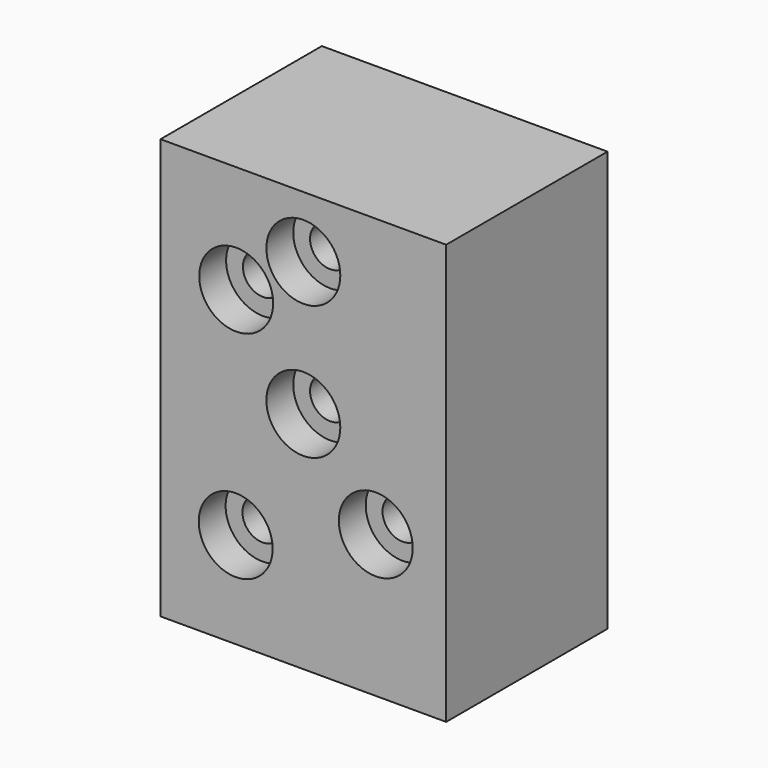
from build123d import *

# Parameters (mm, degrees)
F2_W           = 17
F2_H           = 12
F3_DEPTH       = 25
F5_D           = 2.4
F5_DEPTH       = 12
F5_CBORE_D     = 4.4
F5_CBORE_DEPTH = 2
F5_TIP         = 0.7210327428


# Not quite as in the source:
# - the program builds the solid bodies; features that only make, move or delete a surface that nothing else refers to are left out


with BuildPart() as f3:
    # F2 (on Top) → F3 (new body)
    with BuildSketch(Plane.XY):
        with Locations((0, 16)):
            Rectangle(F2_W, F2_H)
    extrude(amount=F3_DEPTH)

    # F5
    with Locations(Plane.XZ.offset(-10)):
        with Locations((-3.9957389235, 18.5837522149), (0, 21.3394463062), (0, 13.3731160313), (4.3110894039, 8.4640979767), (-4.0247985162, 5.713914521)):
            CounterBoreHole(F5_D / 2, F5_CBORE_D / 2, F5_CBORE_DEPTH, depth=F5_DEPTH)
            with Locations((0, 0, -(F5_DEPTH + F5_TIP / 2))):  # 118° drill point
                Cone(0, F5_D / 2, F5_TIP, mode=Mode.SUBTRACT)


solid = f3.part
